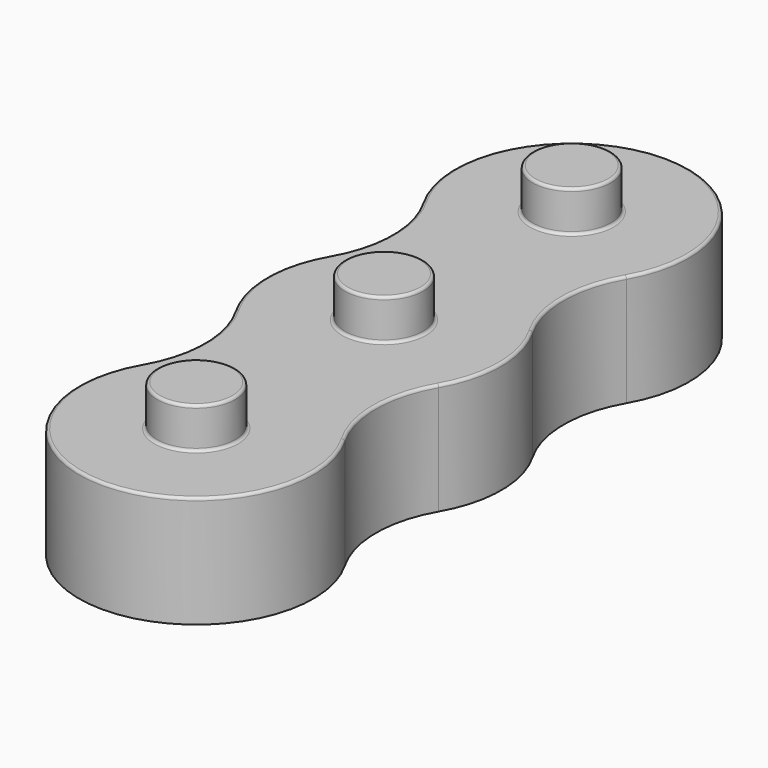
from build123d import *

# Parameters (mm, degrees)
F4_R     = 7.9
F5_DEPTH = 20
F6_DEPTH = 10
F7_R     = 7
F8_DEPTH = 7.3
F9_R     = 0.5


# Not quite as in the source:
# - a feature names something its author has since deleted; it is built from what else it names


with BuildPart() as f5:
    # F4 (on Top) → F5 (new body)
    with BuildSketch(Plane.XY):
        with BuildLine():
            ThreePointArc((18.1865334795, 10.5), (15.3730669589, 21), (18.1865334795, 31.5))
            ThreePointArc((18.1865334795, 31.5), (21, 42), (18.1865334795, 52.5))
            ThreePointArc((18.1865334795, 52.5), (15.3730669589, 63), (18.1865334795, 73.5))
            ThreePointArc((18.1865334795, 73.5), (0, 105), (-18.1865334795, 73.5))
            ThreePointArc((-18.1865334795, 73.5), (-15.3730669589, 63), (-18.1865334795, 52.5))
            ThreePointArc((-18.1865334795, 52.5), (-21, 42), (-18.1865334795, 31.5))
            ThreePointArc((-18.1865334795, 31.5), (-15.3730669589, 21), (-18.1865334795, 10.5))
            ThreePointArc((-18.1865334795, 10.5), (0, -21), (18.1865334795, 10.5))
        make_face()
        Circle(F4_R, mode=Mode.SUBTRACT)
        with Locations((0, 42)):
            Circle(F4_R, mode=Mode.SUBTRACT)
        with Locations((0, 84)):
            Circle(F4_R, mode=Mode.SUBTRACT)
        with Locations((0, 42)):
            Circle(F4_R)
        Circle(F4_R)
        with Locations((0, 84)):
            Circle(F4_R)
    extrude(amount=F5_DEPTH)

    # F4 (on Top) → F6 (cut)
    with BuildSketch(Plane.XY):
        with Locations((0, 42)):
            Circle(F4_R)
        Circle(F4_R)
        with Locations((0, 84)):
            Circle(F4_R)
    extrude(amount=F6_DEPTH, mode=Mode.SUBTRACT)

    # F7 (on face) → F8 (join)
    with BuildSketch(Plane.XY.offset(20)):
        Circle(F7_R)
        with Locations((0, 42)):
            Circle(F7_R)
        with Locations((0, 84)):
            Circle(F7_R)
    extrude(amount=F8_DEPTH)

    # F9
    f9_edges = [f5.edges().sort_by_distance(p)[0] for p in [
        (-7, 0, 27.3),
        (-7.9, 42, 0),
        (-7.9, 42, 10),
        (-7.9, 0, 0),
        (-7.9, 0, 10),
        (-7, 42, 27.3),
        (-7, 42, 20),
        (21, 42, 20),
        (-7, 84, 27.3),
        (-7, 84, 20),
        (-7.9, 84, 10),
        (-7.9, 84, 0),
        (-7, 0, 20),
    ]]
    fillet(f9_edges, radius=F9_R)


solid = f5.part
